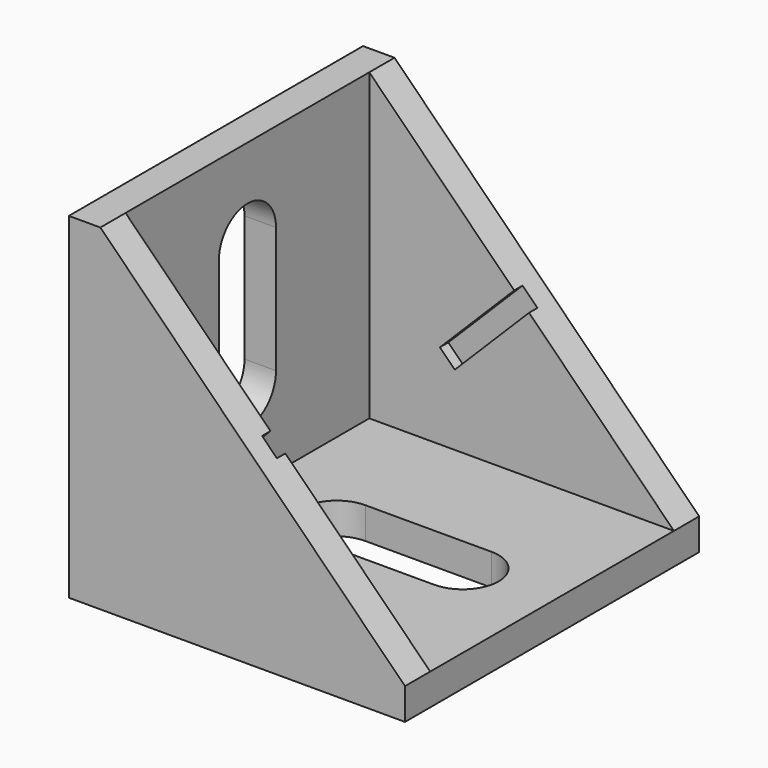
from build123d import *

# Parameters (mm, degrees)
F1_DEPTH  = 35
F2_T      = 3
F4_DEPTH  = 3
F6_DEPTH  = 3
F8_DEPTH  = 1
F10_DEPTH = 1


# Not quite as in the source:
# - a shell that OpenCascade refuses in one call is made with other operations: the cavity is built on its own and cut out


with BuildPart() as f1:
    # F0 (on Front) → F1 (new body)
    with BuildSketch(Plane.XZ):
        Polygon((0, 32), (0, 0), (32, 0), (32, 3), (3, 32), align=None)
    extrude(amount=F1_DEPTH)

    # F2: shell of thickness 3, made by hand


with BuildPart() as f2_core1:
    # F2_t2: copy of F1
    add(f1.part)

    # the walls: a layer under each face that stays
    f2_faces = [f2_core1.faces().sort_by_distance(p)[0] for p in [
        (0, -17.5, 16),
        (16, -17.5, 0),
        (16, 0, 16),
        (16, -35, 16),
    ]]
    thicken(f2_faces, amount=-F2_T, mode=Mode.SUBTRACT)


with BuildPart() as f1_1:
    add(f1.part)

    # what is left inside the walls is the cavity
    f2_cavity = [f2_core1.part.solids().sort_by_distance(p)[0] for p in [
        (17.478787, -22.333333, 17.478787),
    ]]
    add(f2_cavity, mode=Mode.SUBTRACT)

    # F3 (on face) → F4 (cut)
    with BuildSketch(Plane.XY.offset(3)):
        with BuildLine():
            Line((11.5, -20.9), (23.5, -20.9))
            ThreePointArc((23.5, -20.9), (26.9, -17.5), (23.5, -14.1))
            Line((23.5, -14.1), (11.5, -14.1))
            ThreePointArc((11.5, -14.1), (8.1, -17.5), (11.5, -20.9))
        make_face()
    extrude(amount=-F4_DEPTH, mode=Mode.SUBTRACT)

    # F5 (on face) → F6 (cut)
    with BuildSketch(Plane.YZ.offset(3)):
        with BuildLine():
            Line((-14.1, 11.5), (-14.1, 23.5))
            ThreePointArc((-14.1, 23.5), (-17.5, 26.9), (-20.9, 23.5))
            Line((-20.9, 23.5), (-20.9, 11.5))
            ThreePointArc((-20.9, 11.5), (-17.5, 8.1), (-14.1, 11.5))
        make_face()
    extrude(amount=-F6_DEPTH, mode=Mode.SUBTRACT)

    # F7 (on face) → F8 (cut)
    with BuildSketch(Plane.XZ.offset(3)):
        Polygon((11.1360389693, 9.7218254069), (18.2071067812, 16.7928932188), (16.7928932188, 18.2071067812), (9.7218254069, 11.1360389693), align=None)
    extrude(amount=-F8_DEPTH, mode=Mode.SUBTRACT)

    # F9 (on face) → F10 (cut)
    with BuildSketch(Plane(origin=(0, -32, 0), x_dir=(-1, 0, 0), z_dir=(0, 1, 0))):
        Polygon((-16.7928932188, 18.2071067812), (-18.2071067812, 16.7928932188), (-11.1360389693, 9.7218254069), (-9.7218254069, 11.1360389693), align=None)
    extrude(amount=-F10_DEPTH, mode=Mode.SUBTRACT)


solid = f1_1.part
